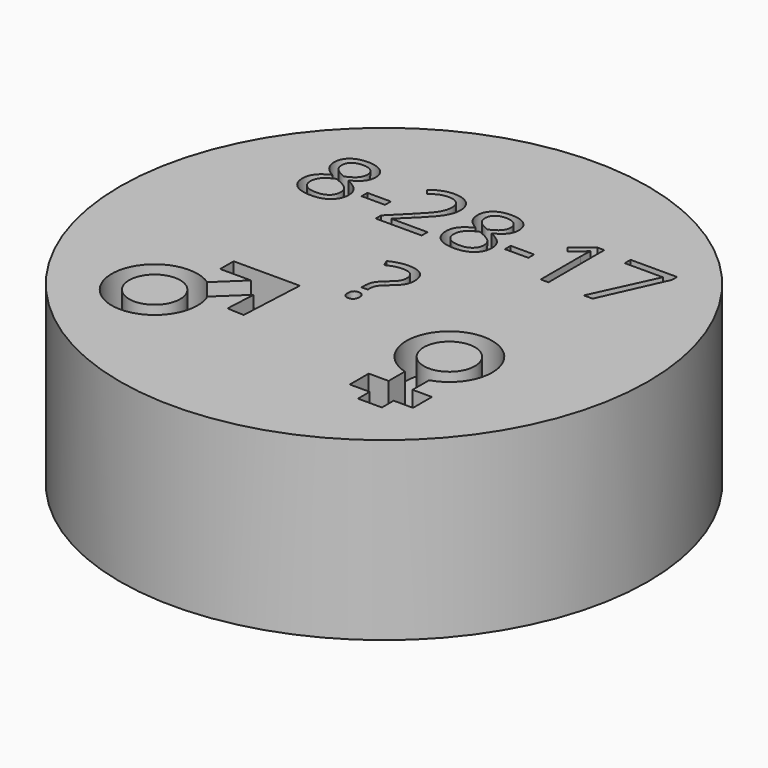
from build123d import *

# Parameters (mm, degrees)
F0_R         = 38.1
F2_DEPTH     = 25.4
F1_R         = 3.6896376877
F3_DEPTH     = 5.0292
F1_W         = 2.7924298106
F1_H         = 3.4081772901
F1_W_2       = 2.8687460604
F4_DEPTH     = 5.08
F1_TEXT_SIZE = 14.1111111111
F5_DEPTH     = 10.16


# Not quite as in the source:
# - Text() gives the source's letters only with a copy of the font that has no kerning and outlines rounded to 1/6400 em; it was checked with that copy


with BuildPart() as f2:
    # F0 (on Top) → F2 (new body)
    with BuildSketch(Plane.XY):
        Circle(F0_R)
    extrude(amount=-F2_DEPTH)

    # F1 (on Top) → F3 (cut)
    with BuildSketch(Plane.XY):
        with BuildLine():
            ThreePointArc((-15.8346386516, -12.0925974171), (-24.7837394896, -20.1087807048), (-13.1237367798, -17.212241888))
            ThreePointArc((-13.1237367798, -17.212241888), (-13.2450616645, -15.9927223548), (-13.604280176, -14.8210100691))
            ThreePointArc((-13.604280176, -14.8210100691), (-14.521187103, -13.2947247671), (-15.8346386516, -12.0925974171))
        make_face()
        with Locations((-19.31351237, -17.212241888)):
            Circle(F1_R, mode=Mode.SUBTRACT)
        with BuildLine():
            ThreePointArc((-15.8346386516, -12.0925974171), (-14.521187103, -13.2947247671), (-13.604280176, -14.8210100691))
            Line((-13.604280176, -14.8210100691), (-9.8207795178, -11.2201712741))
            Line((-9.8207795178, -11.2201712741), (-10.0407487962, -15.6637203669))
            Line((-10.0407487962, -15.6637203669), (-7.6208842235, -15.7835110686))
            Line((-7.6208842235, -15.7835110686), (-7.1490389232, -6.2518720515))
            Line((-7.1490389232, -6.2518720515), (-16.6923496872, -6.2518720515))
            Line((-16.6923496872, -6.2518720515), (-16.6923496872, -8.6746998131))
            Line((-16.6923496872, -8.6746998131), (-12.2433593497, -8.6746998131))
            Line((-12.2433593497, -8.6746998131), (-15.8346386516, -12.0925974171))
        make_face()
    extrude(amount=-F3_DEPTH, mode=Mode.SUBTRACT)

    # F1 (on Top) → F4 (cut)
    with BuildSketch(Plane.XY):
        with BuildLine():
            ThreePointArc((18.6350776911, -15.1603101052), (21.8003810485, -12.9227056723), (23.0141584079, -9.2412978623))
            ThreePointArc((23.0141584079, -9.2412978623), (13.0753703582, -4.3160336626), (15.1759978535, -15.2075486839))
            ThreePointArc((15.1759978535, -15.2075486839), (16.9089049892, -15.4304963451), (18.6350776911, -15.1603101052))
        make_face()
        with Locations((16.8243828177, -9.2412978623)):
            Circle(F1_R, mode=Mode.SUBTRACT)
        Polygon((18.6350776911, -18.1394499219), (15.1759978535, -18.1394499219), (15.1759978535, -21.547627212), (15.1759978535, -23.6694094865), (18.6350776911, -23.6694094865), (18.6350776911, -21.547627212), align=None)
        with BuildLine():
            ThreePointArc((18.6350776911, -15.1603101052), (16.9089049892, -15.4304963451), (15.1759978535, -15.2075486839))
            Line((15.1759978535, -15.2075486839), (15.1759978535, -18.1394499219))
            Line((15.1759978535, -18.1394499219), (18.6350776911, -18.1394499219))
            Line((18.6350776911, -18.1394499219), (18.6350776911, -15.1603101052))
        make_face()
        with Locations((20.0312925964, -19.8435385669)):
            Rectangle(F1_W, F1_H)
        with Locations((13.7416248232, -19.8435385669)):
            Rectangle(F1_W_2, F1_H)
    extrude(amount=-F4_DEPTH, mode=Mode.SUBTRACT)

    # F1 (on Top) → F5 (cut)
    with BuildSketch(Plane.XY):
        with Locations((-23.9986210812, 11.8862119027)):
            Text('8-28-17', F1_TEXT_SIZE, font='Open Sans', text_align=(TextAlign.LEFT, TextAlign.BOTTOM))
        with Locations((-3.4608658118, -4.9900372978)):
            Text('?', F1_TEXT_SIZE, font='Open Sans', text_align=(TextAlign.LEFT, TextAlign.BOTTOM))
    extrude(amount=-F5_DEPTH, mode=Mode.SUBTRACT)


solid = f2.part
